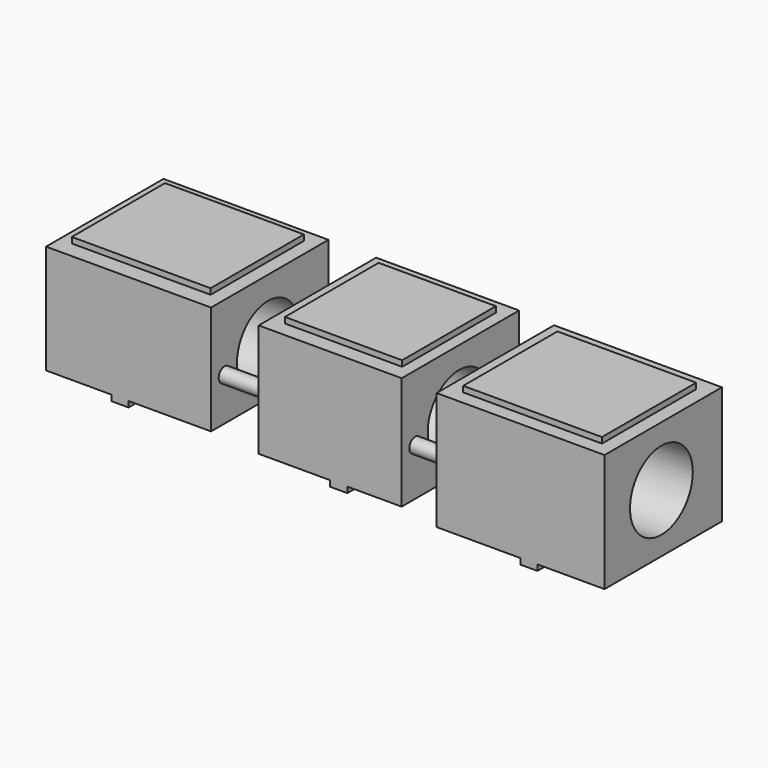
from build123d import *

# Parameters (mm, degrees)
F0_W      = 29.0683805943
F0_H      = 20.4342091456
F1_DEPTH  = 25.4
F2_W      = 24.7512962669
F2_H      = 19.5707976818
F3_DEPTH  = 25.4
F4_W      = 28.5577499308
F4_H      = 18.8771598041
F5_DEPTH  = 25.4
F6_R      = 6.7924602883
F7_DEPTH  = 120
F8_R      = 6.7093285456
F9_DEPTH  = 127
F10_R     = 6.7620138493
F11_DEPTH = 127
F14_R     = 1.27
F15_DEPTH = 50.8
F16_W     = 2.930296585
F16_H     = 25.4
F17_DEPTH = 1
F18_W     = 2.979490906
F18_H     = 25.4
F19_DEPTH = 1
F20_W     = 2.921
F20_H     = 25.4
F21_DEPTH = 1
F22_W     = 24.0344592603
F22_H     = 20.1717780437
F23_DEPTH = 1
F24_W     = 20.2946
F24_H     = 20.2831223141
F25_DEPTH = 1
F26_W     = 24.0173116326
F26_H     = 20.3940093052
F27_DEPTH = 1


# Not quite as in the source:
# - the program builds the solid bodies; features that only make, move or delete a surface that nothing else refers to are left out


with BuildPart() as f1:
    # F0 (on Front) → F1 (new body)
    with BuildSketch(Plane.XZ):
        with Locations((56.9855421782, 24.463489186)):
            Rectangle(F0_W, F0_H)
    extrude(amount=F1_DEPTH)

    # F6 (on face) → F7 (cut)
    with BuildSketch(Plane.YZ.offset(71.5197324753)):
        with Locations((-13.0951609462, 24.3195872754)):
            Circle(F6_R)
    extrude(amount=-F7_DEPTH, mode=Mode.SUBTRACT)

    # F20 (on face) → F21 (join)
    with BuildSketch(Plane(origin=(0, 0, 14.2463846132), x_dir=(1, 0, 0), z_dir=(0, 0, -1))):
        with Locations((58.4460421782, 12.7)):
            Rectangle(F20_W, F20_H)
    extrude(amount=F21_DEPTH)

    # F26 (on face) → F27 (join)
    with BuildSketch(Plane.XY.offset(34.6805937588)):
        with Locations((57.1457631886, -12.8093227977)):
            Rectangle(F26_W, F26_H)
    extrude(amount=F27_DEPTH)


with BuildPart() as f3:
    # F2 (on Front) → F3 (new body)
    with BuildSketch(Plane.XZ):
        with Locations((24.0317806602, 25.1830033958)):
            Rectangle(F2_W, F2_H)
    extrude(amount=F3_DEPTH)

    # F10 (on face) → F11 (cut)
    with BuildSketch(Plane(origin=(11.6561325267, 0, 0), x_dir=(0, -1, 0), z_dir=(-1, 0, 0))):
        with Locations((12.9995224997, 24.4275722653)):
            Circle(F10_R)
    extrude(amount=-F11_DEPTH, mode=Mode.SUBTRACT)

    # F18 (on face) → F19 (join)
    with BuildSketch(Plane(origin=(0, 0, 15.3976045549), x_dir=(1, 0, 0), z_dir=(0, 0, -1))):
        with Locations((25.5215261132, 12.7)):
            Rectangle(F18_W, F18_H)
    extrude(amount=F19_DEPTH)

    # F24 (on face) → F25 (join)
    with BuildSketch(Plane.XY.offset(34.9684022367)):
        with Locations((24.2186706414, -12.6129478449)):
            Rectangle(F24_W, F24_H)
    extrude(amount=F25_DEPTH)


with BuildPart() as f5:
    # F4 (on Front) → F5 (new body)
    with BuildSketch(Plane.XZ):
        with Locations((-10.8705963939, 25.5685206503)):
            Rectangle(F4_W, F4_H)
    extrude(amount=F5_DEPTH)

    # F8 (on face) → F9 (cut)
    with BuildSketch(Plane(origin=(-25.1494713593, 0, 0), x_dir=(0, -1, 0), z_dir=(-1, 0, 0))):
        with Locations((13.0775934085, 24.3113916367)):
            Circle(F8_R)
    extrude(amount=-F9_DEPTH, mode=Mode.SUBTRACT)

    # F16 (on face) → F17 (join)
    with BuildSketch(Plane(origin=(0, 0, 16.1299407482), x_dir=(1, 0, 0), z_dir=(0, 0, -1))):
        with Locations((-12.3357446864, 12.7)):
            Rectangle(F16_W, F16_H)
    extrude(amount=F17_DEPTH)

    # F22 (on face) → F23 (join)
    with BuildSketch(Plane.XY.offset(35.0071005523)):
        with Locations((-10.9888649895, -12.4317585723)):
            Rectangle(F22_W, F22_H)
    extrude(amount=F23_DEPTH)


with BuildPart() as f15:
    # F14 (on face) → F15 (new body)
    with BuildSketch(Plane(origin=(42.451351881, 0, 0), x_dir=(0, -1, 0), z_dir=(-1, 0, 0))):
        with Locations((22.4789213389, 23.6016716808)):
            Circle(F14_R)
    extrude(amount=F15_DEPTH)


solid = Compound([f1.part, f3.part, f5.part, f15.part])
